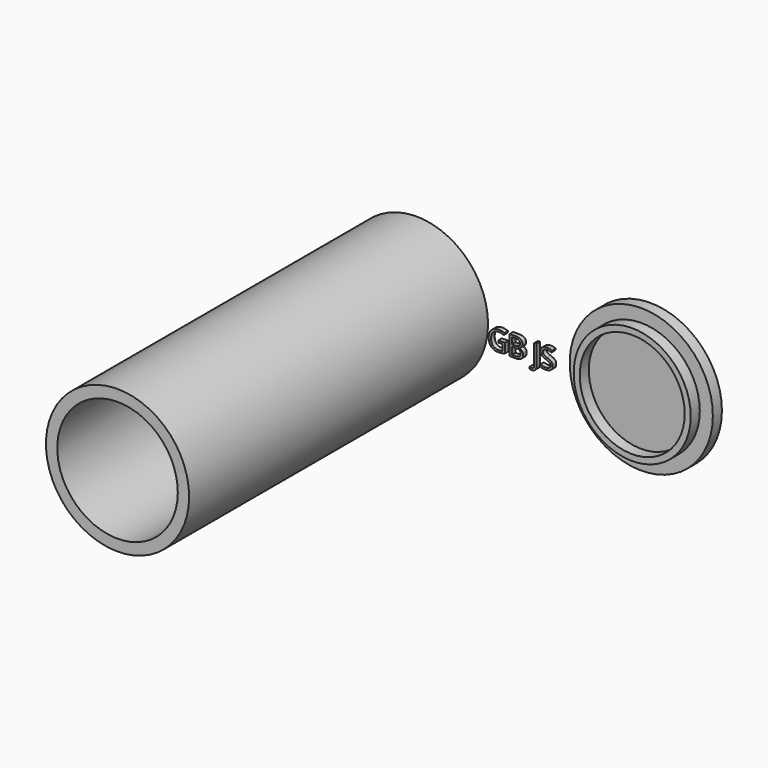
from build123d import *

# Parameters (mm, degrees)
F0_R         = 47.4
F0_R_2       = 39.9
F1_DEPTH     = 239.9
F3_R         = 47.4
F4_DEPTH     = 7.5
F5_R         = 38.75
F5_R_2       = 34.75
F6_DEPTH     = 7.5
F7_SCALE     = 0.5
F8_SCALE     = 0.5
F9_TEXT_SIZE = 18.0772725596
F10_DEPTH    = 3
F11_SCALE    = 0.5


# Not quite as in the source:
# - Text() gives the source's letters only with a copy of the font that has no kerning and outlines rounded to 1/6400 em; it was checked with that copy


with BuildPart() as f1:
    # F0 (on Front) → F1 (new body)
    with BuildSketch(Plane.XZ):
        Circle(F0_R)
        Circle(F0_R_2, mode=Mode.SUBTRACT)
    extrude(amount=F1_DEPTH)

    # F3 (on offset) → F4 (join)
    with BuildSketch(Plane.XZ.offset(-7.5)):
        Circle(F3_R)
    extrude(amount=F4_DEPTH)


with BuildPart() as f4:
    # F3 (on offset) → F4, piece 2 (new body)
    with BuildSketch(Plane.XZ.offset(-7.5)):
        with Locations((154.8447161913, 0)):
            Circle(F3_R)
    extrude(amount=F4_DEPTH)

    # F5 (on face) → F6 (join)
    with BuildSketch(Plane.XZ):
        with Locations((154.8447161913, 0)):
            Circle(F5_R)
        with Locations((154.8447161913, 0)):
            Circle(F5_R_2, mode=Mode.SUBTRACT)
    extrude(amount=F6_DEPTH)


with BuildPart() as f1_1:
    # F7: moved
    add(f1.part.scale(F7_SCALE))


with BuildPart() as f4_1:
    # F8: moved
    add(f4.part.scale(F8_SCALE))


with BuildPart() as f10:
    # F9 (on face) → F10 (new body)
    with BuildSketch(Plane.XZ):
        with Locations((55.1042929292, -6.9968495518)):
            Text('GB JS', F9_TEXT_SIZE, font='Open Sans', text_align=(TextAlign.LEFT, TextAlign.BOTTOM))
    extrude(amount=F10_DEPTH)


with BuildPart() as f10_1:
    # F11: moved
    add(f10.part.scale(F11_SCALE))


solid = Compound([f1_1.part, f4_1.part, f10_1.part])
